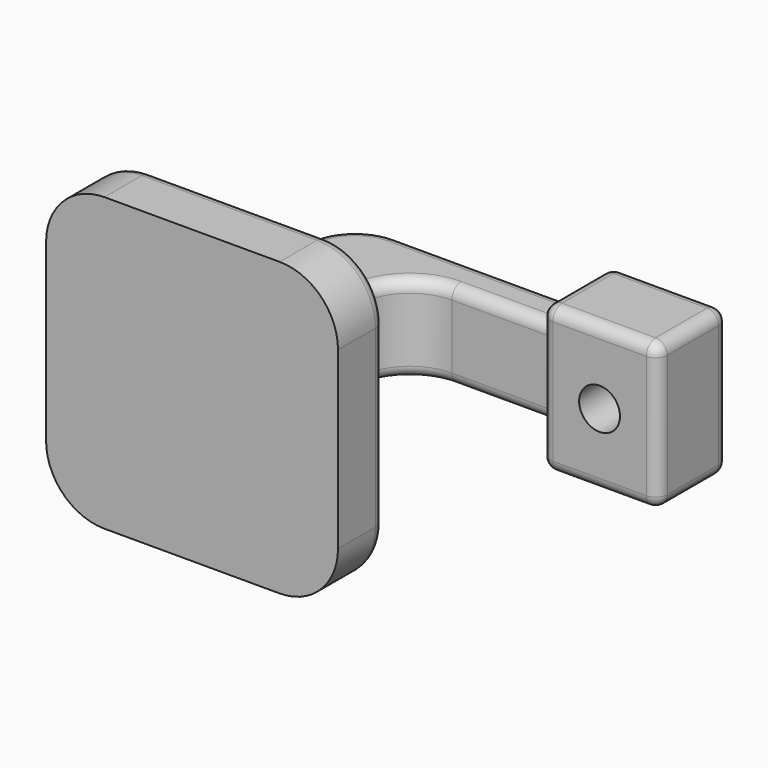
from build123d import *

# Parameters (mm, degrees)
F1_DEPTH = 25
F2_DEPTH = 7.5
F3_DEPTH = 12.5
F4_R     = 10
F5_F1_R  = 2
F5_F2_R  = 2
F6_R     = 3.5
F7_DEPTH = 15
F8_R     = 1.99999


# Not quite as in the source:
# - a fillet or chamfer is up to 0.001 mm smaller than in the source, because OpenCascade refuses the exact size


with BuildPart() as f1:
    # F0 (on Top) → F1 (new body, symmetric)
    with BuildSketch(Plane.XY):
        Polygon((-32.5, 5), (-50, 5), (-50, -5), (0, -5), (0, 5), (-17.5, 5), align=None)
    extrude(amount=F1_DEPTH, both=True)

    # F0 (on Top) → F2 (join, symmetric)
    with BuildSketch(Plane.XY):
        with BuildLine():
            Line((-32.5, 28), (-32.5, 5))
            Line((-32.5, 5), (-17.5, 5))
            Line((-17.5, 5), (-17.5, 21))
            ThreePointArc((-17.5, 21), (-14.8639610307, 27.3639610307), (-8.5, 30))
            Line((-8.5, 30), (10, 30))
            Line((10, 30), (10, 37))
            Line((10, 37), (-23.5, 37))
            ThreePointArc((-23.5, 37), (-29.8639610307, 34.3639610307), (-32.5, 28))
        make_face()
    extrude(amount=F2_DEPTH, both=True)

    # F0 (on Top) → F3 (join, symmetric)
    with BuildSketch(Plane.XY):
        Polygon((10, 41), (10, 37), (10, 30), (10, 26), (30, 26), (30, 41), align=None)
    extrude(amount=F3_DEPTH, both=True)

    # F4
    f4_edges = [f1.edges().sort_by_distance(p)[0] for p in [
        (-50, 0, 25),
        (0, 0, 25),
        (0, 0, -25),
        (-50, 0, -25),
    ]]
    fillet(f4_edges, radius=F4_R)

    # F5: fillet of radius 2 on 26 edges, made by hand

    # F5_f1
    f5_f1_edges = [f1.edges().sort_by_distance(p)[0] for p in [
        (0.75, 30, 7.5),
        (-6.75, 37, 7.5),
        (-29.8639610307, 34.3639610307, 7.5),
        (-32.5, 16.5, 7.5),
        (-17.5, 13, 7.5),
        (-14.8639610307, 27.3639610307, 7.5),
        (0.75, 30, -7.5),
        (-6.75, 37, -7.5),
        (-29.8639610307, 34.3639610307, -7.5),
        (-32.5, 16.5, -7.5),
        (-17.5, 13, -7.5),
        (-14.8639610307, 27.3639610307, -7.5),
        (-50, 5, 0),
        (-47.0710678119, 5, -22.0710678119),
        (-47.0710678119, 5, 22.0710678119),
        (-25, 5, -25),
        (-25, 5, 25),
        (-2.9289321881, 5, -22.0710678119),
        (-2.9289321881, 5, 22.0710678119),
        (0, 5, 0),
    ]]
    fillet(f5_f1_edges, radius=F5_F1_R)

    # F5_f2
    f5_f2_edges = [f1.edges().sort_by_distance(p)[0] for p in [
        (10, 33.5, 7.5),
        (-25, 5, 7.5),
        (10, 33.5, -7.5),
        (-25, 5, -7.5),
        (-17.5, 5, 0),
        (-32.5, 5, 0),
        (-31.9142135624, 5, -6.9142135624),
        (-31.9142135624, 5, 6.9142135624),
        (-18.0857864376, 5, 6.9142135624),
        (-18.0857864376, 5, -6.9142135624),
        (10, 30.5857864376, -6.9142135624),
        (10, 36.4142135624, -6.9142135624),
        (10, 30.5857864376, 6.9142135624),
        (10, 36.4142135624, 6.9142135624),
    ]]
    fillet(f5_f2_edges, radius=F5_F2_R)

    # F6 (on face) → F7 (cut, through all)
    with BuildSketch(Plane(origin=(0, 41, 0), x_dir=(-1, 0, 0), z_dir=(0, 1, 0))):
        with Locations((-20, 0)):
            Circle(F6_R)
    extrude(amount=-F7_DEPTH, mode=Mode.SUBTRACT)

    # F8 (radius 2 in the source; OpenCascade refuses exactly that, so slightly less here)
    f8_edges = [f1.edges().sort_by_distance(p)[0] for p in [
        (10, 33.5, -12.5),
        (20, 26, -12.5),
        (30, 33.5, -12.5),
        (20, 41, -12.5),
        (10, 33.5, 12.5),
        (20, 26, 12.5),
        (30, 33.5, 12.5),
        (20, 41, 12.5),
        (30, 41, 0),
        (30, 26, 0),
        (10, 41, 0),
        (10, 26, 0),
    ]]
    fillet(f8_edges, radius=F8_R)


solid = f1.part
